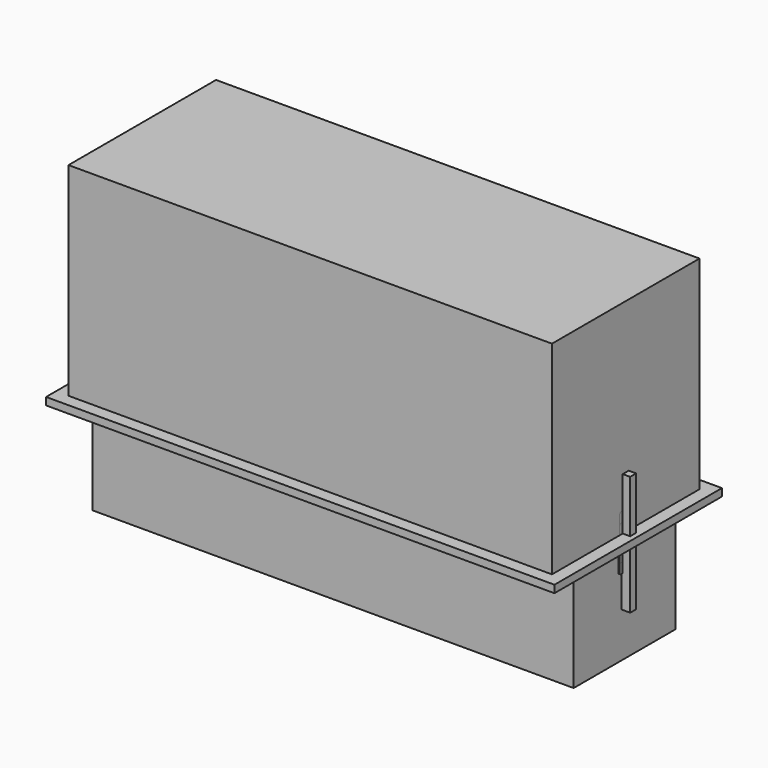
from build123d import *

# Parameters (mm, degrees)
F4_W      = 1231.9
F4_H      = 469.9
F5_DEPTH  = 536.575
F6_W      = 914.4
F6_H      = 317.5
F7_DEPTH  = 406.4
F9_W      = 1295.4
F9_H      = 533.4
F10_DEPTH = 19.05
F13_DEPTH = 196.85
F14_DEPTH = 615.95
F15_DEPTH = 196.85
F16_DEPTH = 615.95
F18_DEPTH = 273.05
F19_DEPTH = 273.05
F20_DEPTH = 273.05
F22_DEPTH = 546.1
F23_W     = 19.05
F23_H     = 152.4
F24_DEPTH = 234.95
F25_DEPTH = 635
F27_W     = 19.05
F27_H     = 469.9
F28_DEPTH = 31.75
F29_DEPTH = 73.025
F31_DEPTH = 57.15
F32_W     = 425.45
F32_H     = 463.55
F33_DEPTH = 9.525
F34_W     = 336.55
F34_H     = 463.55
F35_DEPTH = 9.525
F37_W     = 1225.55
F37_H     = 533.4
F38_DEPTH = 161.925
F39_W     = 19.05
F39_H     = 304.8
F40_DEPTH = 234.95
F41_W     = 19.05
F41_H     = 76.2
F42_DEPTH = 635
F43_DEPTH = 635
F44_W     = 114.3
F44_H     = 152.4
F45_DEPTH = 9.525
F46_W     = 146.05
F46_H     = 152.4
F47_DEPTH = 9.525
F48_W     = 425.45
F48_H     = 146.05
F49_DEPTH = 9.525
F50_W     = 19.05
F50_H     = 25.4
F51_DEPTH = 615.95


with BuildPart() as f5:
    # F4 (on Top) → F5 (new body)
    with BuildSketch(Plane.XY):
        Rectangle(F4_W, F4_H)
    extrude(amount=F5_DEPTH)


with BuildPart() as f7:
    # F6 (on Top) → F7 (new body)
    with BuildSketch(Plane.XY):
        Rectangle(F6_W, F6_H)
    extrude(amount=F7_DEPTH)


with BuildPart() as f10:
    # F9 (on Top) → F10 (new body)
    with BuildSketch(Plane.XY):
        Rectangle(F9_W, F9_H)
    extrude(amount=F10_DEPTH)


with BuildPart() as f13:
    # F12 (on Right) → F13 (new body, symmetric)
    with BuildSketch(Plane.YZ):
        with BuildLine():
            ThreePointArc((19.05, 66.675), (18.1200640303, 68.9200640303), (15.875, 69.85))
            Line((15.875, 69.85), (-15.875, 69.85))
            ThreePointArc((-15.875, 69.85), (-18.1200640303, 68.9200640303), (-19.05, 66.675))
            Line((-19.05, 66.675), (-19.05, -66.675))
            ThreePointArc((-19.05, -66.675), (-18.1200640303, -68.9200640303), (-15.875, -69.85))
            Line((-15.875, -69.85), (15.875, -69.85))
            ThreePointArc((15.875, -69.85), (18.1200640303, -68.9200640303), (19.05, -66.675))
            Line((19.05, -66.675), (19.05, 66.675))
        make_face()
    extrude(amount=F13_DEPTH, both=True)


with BuildPart() as f14:
    # F12 (on Right) → F14 (new body, symmetric)
    with BuildSketch(Plane.YZ):
        with BuildLine():
            ThreePointArc((19.05, 66.675), (18.1200640303, 68.9200640303), (15.875, 69.85))
            Line((15.875, 69.85), (-15.875, 69.85))
            ThreePointArc((-15.875, 69.85), (-18.1200640303, 68.9200640303), (-19.05, 66.675))
            Line((-19.05, 66.675), (-19.05, -66.675))
            ThreePointArc((-19.05, -66.675), (-18.1200640303, -68.9200640303), (-15.875, -69.85))
            Line((-15.875, -69.85), (15.875, -69.85))
            ThreePointArc((15.875, -69.85), (18.1200640303, -68.9200640303), (19.05, -66.675))
            Line((19.05, -66.675), (19.05, 66.675))
        make_face()
    extrude(amount=F14_DEPTH, both=True)


with BuildPart() as f15:
    # F11 (on Right) → F15 (new body, symmetric)
    with BuildSketch(Plane.YZ):
        with BuildLine():
            ThreePointArc((19.05, 41.275), (18.1200640303, 43.5200640303), (15.875, 44.45))
            Line((15.875, 44.45), (-15.875, 44.45))
            ThreePointArc((-15.875, 44.45), (-18.1200640303, 43.5200640303), (-19.05, 41.275))
            Line((-19.05, 41.275), (-19.05, -41.275))
            ThreePointArc((-19.05, -41.275), (-18.1200640303, -43.5200640303), (-15.875, -44.45))
            Line((-15.875, -44.45), (15.875, -44.45))
            ThreePointArc((15.875, -44.45), (18.1200640303, -43.5200640303), (19.05, -41.275))
            Line((19.05, -41.275), (19.05, 41.275))
        make_face()
    extrude(amount=F15_DEPTH, both=True)


with BuildPart() as f16:
    # F11 (on Right) → F16 (new body, symmetric)
    with BuildSketch(Plane.YZ):
        with BuildLine():
            ThreePointArc((19.05, 41.275), (18.1200640303, 43.5200640303), (15.875, 44.45))
            Line((15.875, 44.45), (-15.875, 44.45))
            ThreePointArc((-15.875, 44.45), (-18.1200640303, 43.5200640303), (-19.05, 41.275))
            Line((-19.05, 41.275), (-19.05, -41.275))
            ThreePointArc((-19.05, -41.275), (-18.1200640303, -43.5200640303), (-15.875, -44.45))
            Line((-15.875, -44.45), (15.875, -44.45))
            ThreePointArc((15.875, -44.45), (18.1200640303, -43.5200640303), (19.05, -41.275))
            Line((19.05, -41.275), (19.05, 41.275))
        make_face()
    extrude(amount=F16_DEPTH, both=True)


with BuildPart() as f18:
    # F12 (on Right) → F18 (new body, symmetric)
    with BuildSketch(Plane.YZ):
        with BuildLine():
            ThreePointArc((19.05, 66.675), (18.1200640303, 68.9200640303), (15.875, 69.85))
            Line((15.875, 69.85), (-15.875, 69.85))
            ThreePointArc((-15.875, 69.85), (-18.1200640303, 68.9200640303), (-19.05, 66.675))
            Line((-19.05, 66.675), (-19.05, -66.675))
            ThreePointArc((-19.05, -66.675), (-18.1200640303, -68.9200640303), (-15.875, -69.85))
            Line((-15.875, -69.85), (15.875, -69.85))
            ThreePointArc((15.875, -69.85), (18.1200640303, -68.9200640303), (19.05, -66.675))
            Line((19.05, -66.675), (19.05, 66.675))
        make_face()
    extrude(amount=F18_DEPTH, both=True)


with BuildPart() as f19:
    # F11 (on Right) → F19 (new body, symmetric)
    with BuildSketch(Plane.YZ):
        with BuildLine():
            ThreePointArc((19.05, 41.275), (18.1200640303, 43.5200640303), (15.875, 44.45))
            Line((15.875, 44.45), (-15.875, 44.45))
            ThreePointArc((-15.875, 44.45), (-18.1200640303, 43.5200640303), (-19.05, 41.275))
            Line((-19.05, 41.275), (-19.05, -41.275))
            ThreePointArc((-19.05, -41.275), (-18.1200640303, -43.5200640303), (-15.875, -44.45))
            Line((-15.875, -44.45), (15.875, -44.45))
            ThreePointArc((15.875, -44.45), (18.1200640303, -43.5200640303), (19.05, -41.275))
            Line((19.05, -41.275), (19.05, 41.275))
        make_face()
    extrude(amount=F19_DEPTH, both=True)


with BuildPart() as f20:
    # F11 (on Right) → F20 (new body, symmetric)
    with BuildSketch(Plane.YZ):
        with BuildLine():
            ThreePointArc((19.05, 41.275), (18.1200640303, 43.5200640303), (15.875, 44.45))
            Line((15.875, 44.45), (-15.875, 44.45))
            ThreePointArc((-15.875, 44.45), (-18.1200640303, 43.5200640303), (-19.05, 41.275))
            Line((-19.05, 41.275), (-19.05, -41.275))
            ThreePointArc((-19.05, -41.275), (-18.1200640303, -43.5200640303), (-15.875, -44.45))
            Line((-15.875, -44.45), (15.875, -44.45))
            ThreePointArc((15.875, -44.45), (18.1200640303, -43.5200640303), (19.05, -41.275))
            Line((19.05, -41.275), (19.05, 41.275))
        make_face()
    extrude(amount=F20_DEPTH, both=True)

    # F21 (on face) → F22 (cut, through all)
    with BuildSketch(Plane(origin=(-273.05, 0, 0), x_dir=(0, -1, 0), z_dir=(-1, 0, 0))):
        with BuildLine():
            Line((-19.05, 41.275), (-19.05, 19.05))
            Line((-19.05, 19.05), (19.05, 19.05))
            Line((19.05, 19.05), (19.05, 41.275))
            ThreePointArc((19.05, 41.275), (18.1200640303, 43.5200640303), (15.875, 44.45))
            Line((15.875, 44.45), (-15.875, 44.45))
            ThreePointArc((-15.875, 44.45), (-18.1200640303, 43.5200640303), (-19.05, 41.275))
        make_face()
    extrude(amount=-F22_DEPTH, mode=Mode.SUBTRACT)


with BuildPart() as f24:
    # F23 (on Right) → F24 (new body, symmetric)
    with BuildSketch(Plane.YZ):
        Rectangle(F23_W, F23_H)
    extrude(amount=F24_DEPTH, both=True)


with BuildPart() as f25:
    # F23 (on Right) → F25 (new body, symmetric)
    with BuildSketch(Plane.YZ):
        Rectangle(F23_W, F23_H)
    extrude(amount=F25_DEPTH, both=True)


with BuildPart() as f28:
    # F27 (on Front) → F28 (new body, symmetric)
    with BuildSketch(Plane.XZ):
        Rectangle(F27_W, F27_H)
    extrude(amount=F28_DEPTH, both=True)


with BuildPart() as f29:
    # F27 (on Front) → F29 (new body, symmetric)
    with BuildSketch(Plane.XZ):
        Rectangle(F27_W, F27_H)
    extrude(amount=F29_DEPTH, both=True)


with BuildPart() as f31:
    # F27 (on Front) → F31 (new body, symmetric)
    with BuildSketch(Plane.XZ):
        Rectangle(F27_W, F27_H)
    extrude(amount=F31_DEPTH, both=True)


with BuildPart() as f33:
    # F32 (on Front) → F33 (new body, symmetric)
    with BuildSketch(Plane.XZ):
        Rectangle(F32_W, F32_H)
    extrude(amount=F33_DEPTH, both=True)


with BuildPart() as f35:
    # F34 (on Front) → F35 (new body, symmetric)
    with BuildSketch(Plane.XZ):
        Rectangle(F34_W, F34_H)
    extrude(amount=F35_DEPTH, both=True)


with BuildPart() as f38:
    # F37 (on Front) → F38 (new body, symmetric)
    with BuildSketch(Plane.XZ):
        Rectangle(F37_W, F37_H)
    extrude(amount=F38_DEPTH, both=True)


with BuildPart() as f40:
    # F39 (on Right) → F40 (new body, symmetric)
    with BuildSketch(Plane.YZ):
        Rectangle(F39_W, F39_H)
    extrude(amount=F40_DEPTH, both=True)


with BuildPart() as f42:
    # F41 (on Right) → F42 (new body, symmetric)
    with BuildSketch(Plane.YZ):
        Rectangle(F41_W, F41_H)
    extrude(amount=F42_DEPTH, both=True)


with BuildPart() as f43:
    # F39 (on Right) → F43 (new body, symmetric)
    with BuildSketch(Plane.YZ):
        Rectangle(F39_W, F39_H)
    extrude(amount=F43_DEPTH, both=True)


with BuildPart() as f45:
    # F44 (on Front) → F45 (new body, symmetric)
    with BuildSketch(Plane.XZ):
        Rectangle(F44_W, F44_H)
    extrude(amount=F45_DEPTH, both=True)


with BuildPart() as f47:
    # F46 (on Front) → F47 (new body, symmetric)
    with BuildSketch(Plane.XZ):
        Rectangle(F46_W, F46_H)
    extrude(amount=F47_DEPTH, both=True)


with BuildPart() as f49:
    # F48 (on Front) → F49 (new body, symmetric)
    with BuildSketch(Plane.XZ):
        Rectangle(F48_W, F48_H)
    extrude(amount=F49_DEPTH, both=True)


with BuildPart() as f51:
    # F50 (on Right) → F51 (new body, symmetric)
    with BuildSketch(Plane.YZ):
        Rectangle(F50_W, F50_H)
    extrude(amount=F51_DEPTH, both=True)


solid = Compound([f5.part, f7.part, f10.part, f13.part, f14.part, f15.part, f16.part, f18.part, f19.part, f20.part, f24.part, f25.part, f28.part, f29.part, f31.part, f33.part, f35.part, f38.part, f40.part, f42.part, f43.part, f45.part, f47.part, f49.part, f51.part])
